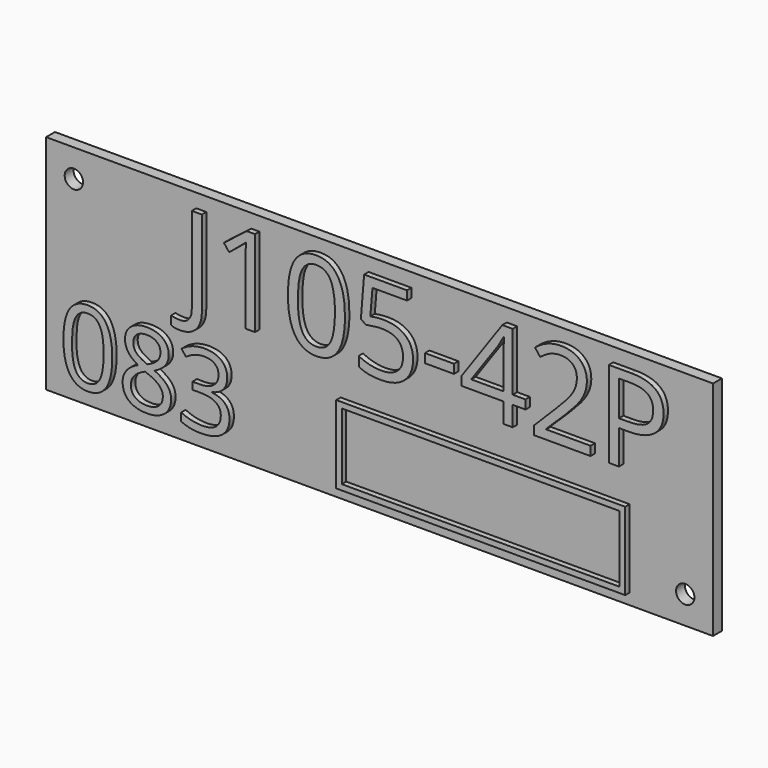
from build123d import *

# Parameters (mm, degrees)
F0_W         = 120
F0_H         = 40
F1_DEPTH     = 2
F3_D         = 3.3
F4_TEXT_SIZE = 21.733388673
F5_DEPTH     = 1
F6_TEXT_SIZE = 18.5894526641
F7_DEPTH     = 1
F8_W         = 52
F8_H         = 14
F8_W_2       = 49.99999962
F8_H_2       = 11.99999962
F9_DEPTH     = 1


# Not quite as in the source:
# - Text() gives the source's letters only with a copy of the font that has no kerning and outlines rounded to 1/6400 em; it was checked with that copy


with BuildPart() as f1:
    # F0 (on Front) → F1 (new body)
    with BuildSketch(Plane.XZ):
        Rectangle(F0_W, F0_H)
    extrude(amount=F1_DEPTH)

    # F3 (through all)
    with Locations(Plane.XZ.offset(2)):
        with Locations((-55, 15), (55, -15)):
            Hole(F3_D / 2)

    # F4 (on face) → F5 (join)
    with BuildSketch(Plane.XZ.offset(2)):
        with Locations((-35, 2)):
            Text('J105-42P', F4_TEXT_SIZE, font='Open Sans', text_align=(TextAlign.LEFT, TextAlign.BOTTOM))
    extrude(amount=F5_DEPTH)

    # F6 (on face) → F7 (join)
    with BuildSketch(Plane.XZ.offset(2)):
        with Locations((-57, -17)):
            Text('083', F6_TEXT_SIZE, font='Open Sans', text_align=(TextAlign.LEFT, TextAlign.BOTTOM))
    extrude(amount=F7_DEPTH)

    # F8 (on face) → F9 (join)
    with BuildSketch(Plane.XZ.offset(2)):
        with Locations((19, -11)):
            Rectangle(F8_W, F8_H)
        with Locations((19, -11)):
            Rectangle(F8_W_2, F8_H_2, mode=Mode.SUBTRACT)
    extrude(amount=F9_DEPTH)


solid = f1.part
